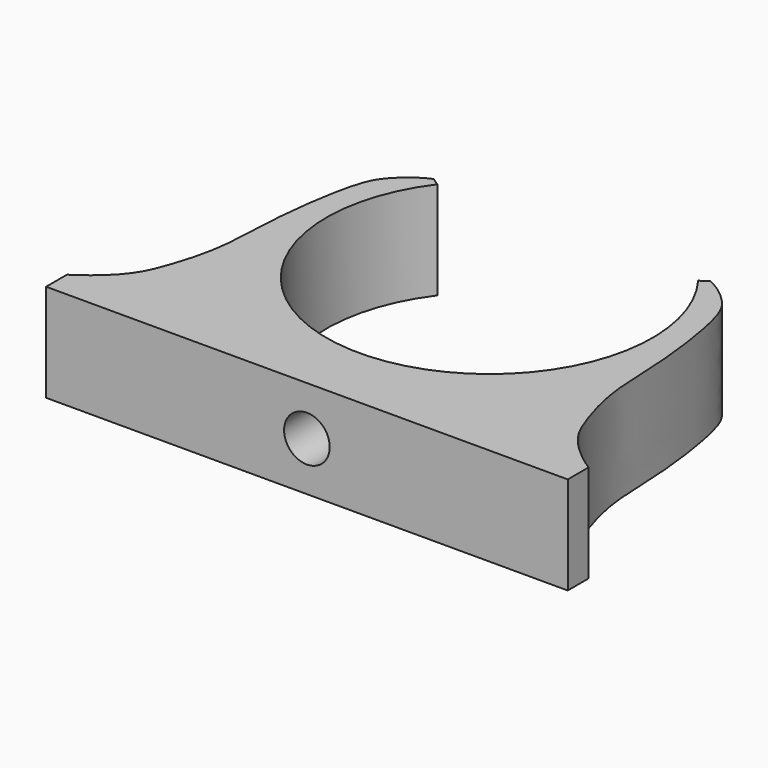
from build123d import *

# Parameters (mm, degrees)
F1_DEPTH = 15
F2_R     = 3.5
F3_DEPTH = 25


with BuildPart() as f1:
    # F0 (on Top) → F1 (new body)
    with BuildSketch(Plane.XY):
        with BuildLine():
            ThreePointArc((20, 50), (22.360679775, 23.8196601125), (0, 10))
            Line((0, 10), (0, 0))
            Line((0, 0), (40, 0))
            Line((40, 0), (40, 4))
            add(Edge.make_bspline(
                [(21.2116204202, 50.796829164), (22.723159163, 50.2030951154), (25.7822546717, 47.7526835762), (27.9001408447, 44.1260945679), (29.8802889933, 31.195596433), (29.7191742065, 21.2106955797), (31.9626402727, 13.6210645558), (34.0110364625, 8.503878025), (38.3847694363, 4.9683936974), (40, 4)],
                knots=[0, 0, 0, 0, 0.1203725941, 0.2286814467, 0.417086039, 0.5893969564, 0.7338405817, 0.8590175959, 1, 1, 1, 1], degree=3))
            Line((21.2116204202, 50.796829164), (20, 50))
        make_face()
        with BuildLine():
            Line((0, 0), (0, 10))
            ThreePointArc((0, 10), (-22.360679775, 23.8196601125), (-20, 50))
            Line((-20, 50), (-21.2116204202, 50.796829164))
            add(Edge.make_bspline(
                [(-21.2116204202, 50.796829164), (-22.723159163, 50.2030951154), (-25.7822546717, 47.7526835762), (-27.9001408447, 44.1260945679), (-29.8802889933, 31.195596433), (-29.7191742065, 21.2106955797), (-31.9626402727, 13.6210645558), (-34.0110364625, 8.503878025), (-38.3847694363, 4.9683936974), (-40, 4)],
                knots=[0, 0, 0, 0, 0.1203725941, 0.2286814467, 0.417086039, 0.5893969564, 0.7338405817, 0.8590175959, 1, 1, 1, 1], degree=3))
            Line((-40, 4), (-40, 0))
            Line((-40, 0), (0, 0))
        make_face()
    extrude(amount=F1_DEPTH)

    # F2 (on face) → F3 (cut)
    with BuildSketch(Plane.XZ):
        with Locations((0, 7.5)):
            Circle(F2_R)
    extrude(amount=-F3_DEPTH, mode=Mode.SUBTRACT)


solid = f1.part
